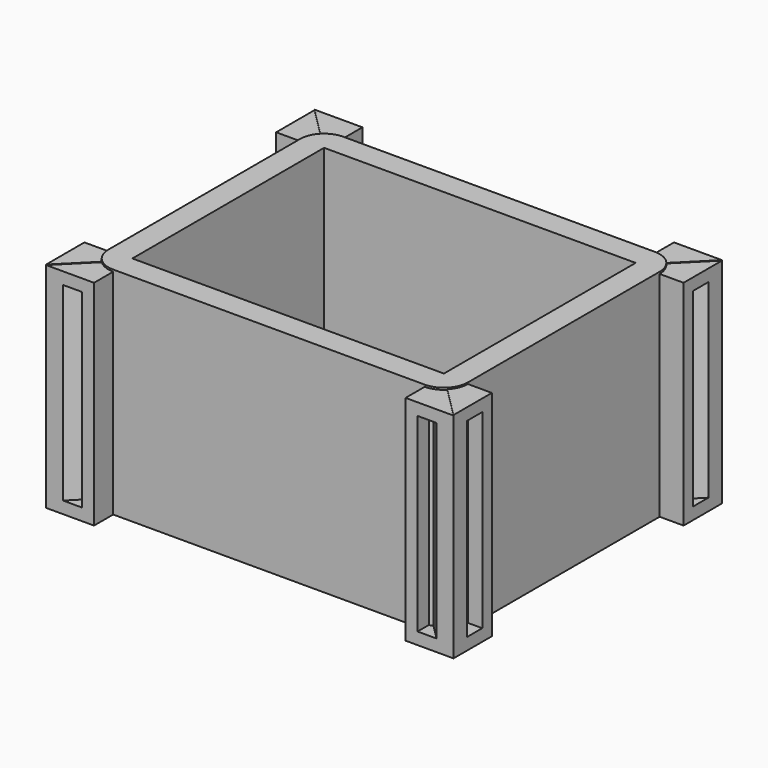
from build123d import *

# Parameters (mm, degrees)
F0_W         = 65
F0_H         = 5
F0_W_2       = 5
F0_H_2       = 50
F1_DEPTH     = 45
F2_DEPTH     = 0.1
F4_DEPTH     = 0.8
F5_DEPTH     = 44.6
F6_DEPTH     = 44.7
F7_T         = -2.5
F7_2_T       = -2.5
F7_3_T       = -2.5
F7_4_T       = -2.5
F7_5_T       = -2.5
F7_6_T       = -2.5
F7_7_T       = -2.5
F7_8_T       = -2.5
F8_TEXT_SIZE = 4.8791821529
F9_DEPTH     = 1


# Not quite as in the source:
# - Text() gives the source's letters only with a copy of the font that has no kerning and outlines rounded to 1/6400 em; it was checked with that copy


with BuildPart() as f1:
    # F0 (on Top) → F1 (new body)
    with BuildSketch(Plane.XY):
        with Locations((0, -27.5)):
            Rectangle(F0_W, F0_H)
        with Locations((0, 27.5)):
            Rectangle(F0_W, F0_H)
        with Locations((35, 0)):
            Rectangle(F0_W_2, F0_H_2)
        with Locations((-35, 0)):
            Rectangle(F0_W_2, F0_H_2)
        with BuildLine():
            Line((36.0355339059, 28.5355339059), (32.5, 25))
            Line((32.5, 25), (37.5, 25))
            ThreePointArc((37.5, 25), (37.1193976626, 26.9134171618), (36.0355339059, 28.5355339059))
        make_face()
        with BuildLine():
            Line((32.5, 30), (32.5, 25))
            Line((32.5, 25), (36.0355339059, 28.5355339059))
            ThreePointArc((36.0355339059, 28.5355339059), (34.4134171618, 29.6193976626), (32.5, 30))
        make_face()
        with BuildLine():
            Line((32.5, -25), (32.5, -30))
            ThreePointArc((32.5, -30), (34.4134171618, -29.6193976626), (36.0355339059, -28.5355339059))
            Line((36.0355339059, -28.5355339059), (32.5, -25))
        make_face()
        with BuildLine():
            Line((32.5, -25), (36.0355339059, -28.5355339059))
            ThreePointArc((36.0355339059, -28.5355339059), (37.1193976626, -26.9134171618), (37.5, -25))
            Line((37.5, -25), (32.5, -25))
        make_face()
        with BuildLine():
            ThreePointArc((-37.5, -25), (-37.1193976626, -26.9134171618), (-36.0355339059, -28.5355339059))
            Line((-36.0355339059, -28.5355339059), (-32.5, -25))
            Line((-32.5, -25), (-37.5, -25))
        make_face()
        with BuildLine():
            ThreePointArc((-36.0355339059, -28.5355339059), (-34.4134171618, -29.6193976626), (-32.5, -30))
            Line((-32.5, -30), (-32.5, -25))
            Line((-32.5, -25), (-36.0355339059, -28.5355339059))
        make_face()
        with BuildLine():
            Line((-36.0355339059, 28.5355339059), (-32.5, 25))
            Line((-32.5, 25), (-32.5, 30))
            ThreePointArc((-32.5, 30), (-34.4134171618, 29.6193976626), (-36.0355339059, 28.5355339059))
        make_face()
        with BuildLine():
            Line((-37.5, 25), (-32.5, 25))
            Line((-32.5, 25), (-36.0355339059, 28.5355339059))
            ThreePointArc((-36.0355339059, 28.5355339059), (-37.1193976626, 26.9134171618), (-37.5, 25))
        make_face()
    extrude(amount=F1_DEPTH)

    # F0 (on Top) → F2 (join)
    with BuildSketch(Plane.XY):
        Rectangle(F0_W, F0_H_2)
    extrude(amount=F2_DEPTH)

    # F3 (on face) → F4 (join)
    with BuildSketch(Plane.XY):
        Polygon((9.8419218215, 7.8486707481), (0, 12.5882904977), (-9.8419218215, 7.8486707481), (-12.2726757728, -2.8011581585), (-5.4618545502, -11.3416578385), (5.4618545502, -11.3416578385), (12.2726757728, -2.8011581585), align=None)
        Polygon((4.0130618095, 14.8103222201), (5.6598507799, 20.3949809074), (1.6467889705, 24.6134713342), (-4.0130618095, 23.2473030736), (-5.6598507799, 17.6626443863), (-1.6467889705, 13.4441539595), align=None)
        Polygon((-15.0811464459, -4.2184904268), (-13.4343574755, 1.3661682606), (-17.447419285, 5.5846586873), (-23.1072700649, 4.2184904268), (-24.7540590353, -1.3661682606), (-20.7409972259, -5.5846586873), align=None)
        Polygon((22.6341824114, -4.2184904268), (24.2809713818, 1.3661682606), (20.2679095724, 5.5846586873), (14.6080587924, 4.2184904268), (12.961269822, -1.3661682606), (16.9743316314, -5.5846586873), align=None)
        Polygon((4.0130618095, -23.7464398195), (5.6598507799, -18.1617811322), (1.6467889705, -13.9432907055), (-4.0130618095, -15.309458966), (-5.6598507799, -20.8941176534), (-1.6467889705, -25.1126080801), align=None)
    extrude(amount=F4_DEPTH)

    # F8 (on face) → F9 (join)
    with BuildSketch(Plane(origin=(0, 30, 0), x_dir=(-1, 0, 0), z_dir=(0, 1, 0))):
        with Locations((-26.7379190773, 13.3689595386)):
            Text('Vote For Harambe 2017', F8_TEXT_SIZE, font='Open Sans', text_align=(TextAlign.LEFT, TextAlign.BOTTOM))
    extrude(amount=F9_DEPTH)


with BuildPart() as f5:
    # F0 (on Top) → F5 (new body)
    with BuildSketch(Plane.XY):
        with BuildLine():
            Line((-42.5, 25), (-37.5, 25))
            ThreePointArc((-37.5, 25), (-37.1193976626, 26.9134171618), (-36.0355339059, 28.5355339059))
            Line((-36.0355339059, 28.5355339059), (-42.5, 35))
            Line((-42.5, 35), (-42.5, 25))
        make_face()
    extrude(amount=F5_DEPTH)

    # F7#8
    f7_8_openings = [f5.faces().sort_by_distance(p)[0] for p in [
        (-42.5, 30, 22.3),
    ]]
    offset(amount=F7_8_T, openings=f7_8_openings)


with BuildPart() as f5b:
    # F0 (on Top) → F5, piece 2 (new body)
    with BuildSketch(Plane.XY):
        with BuildLine():
            Line((-32.5, -35), (-32.5, -30))
            ThreePointArc((-32.5, -30), (-34.4134171618, -29.6193976626), (-36.0355339059, -28.5355339059))
            Line((-36.0355339059, -28.5355339059), (-42.5, -35))
            Line((-42.5, -35), (-32.5, -35))
        make_face()
    extrude(amount=F5_DEPTH)

    # F7
    f7_openings = [f5b.faces().sort_by_distance(p)[0] for p in [
        (-37.5, -35, 22.3),
    ]]
    offset(amount=F7_T, openings=f7_openings)


with BuildPart() as f5c:
    # F0 (on Top) → F5, piece 3 (new body)
    with BuildSketch(Plane.XY):
        with BuildLine():
            ThreePointArc((36.0355339059, 28.5355339059), (37.1193976626, 26.9134171618), (37.5, 25))
            Line((37.5, 25), (42.5, 25))
            Line((42.5, 25), (42.5, 35))
            Line((42.5, 35), (36.0355339059, 28.5355339059))
        make_face()
    extrude(amount=F5_DEPTH)

    # F7#5
    f7_5_openings = [f5c.faces().sort_by_distance(p)[0] for p in [
        (42.5, 30, 22.3),
    ]]
    offset(amount=F7_5_T, openings=f7_5_openings)


with BuildPart() as f5d:
    # F0 (on Top) → F5, piece 4 (new body)
    with BuildSketch(Plane.XY):
        with BuildLine():
            ThreePointArc((36.0355339059, -28.5355339059), (34.4134171618, -29.6193976626), (32.5, -30))
            Line((32.5, -30), (32.5, -35))
            Line((32.5, -35), (42.5, -35))
            Line((42.5, -35), (36.0355339059, -28.5355339059))
        make_face()
    extrude(amount=F5_DEPTH)

    # F7#3
    f7_3_openings = [f5d.faces().sort_by_distance(p)[0] for p in [
        (37.5, -35, 22.3),
    ]]
    offset(amount=F7_3_T, openings=f7_3_openings)


with BuildPart() as f6:
    # F0 (on Top) → F6 (new body)
    with BuildSketch(Plane.XY):
        with BuildLine():
            Line((-42.5, -35), (-36.0355339059, -28.5355339059))
            ThreePointArc((-36.0355339059, -28.5355339059), (-37.1193976626, -26.9134171618), (-37.5, -25))
            Line((-37.5, -25), (-42.5, -25))
            Line((-42.5, -25), (-42.5, -35))
        make_face()
    extrude(amount=F6_DEPTH)

    # F7#2
    f7_2_openings = [f6.faces().sort_by_distance(p)[0] for p in [
        (-42.5, -30, 22.35),
    ]]
    offset(amount=F7_2_T, openings=f7_2_openings)


with BuildPart() as f6b:
    # F0 (on Top) → F6, piece 2 (new body)
    with BuildSketch(Plane.XY):
        with BuildLine():
            ThreePointArc((37.5, -25), (37.1193976626, -26.9134171618), (36.0355339059, -28.5355339059))
            Line((36.0355339059, -28.5355339059), (42.5, -35))
            Line((42.5, -35), (42.5, -25))
            Line((42.5, -25), (37.5, -25))
        make_face()
    extrude(amount=F6_DEPTH)

    # F7#4
    f7_4_openings = [f6b.faces().sort_by_distance(p)[0] for p in [
        (42.5, -30, 22.35),
    ]]
    offset(amount=F7_4_T, openings=f7_4_openings)


with BuildPart() as f6c:
    # F0 (on Top) → F6, piece 3 (new body)
    with BuildSketch(Plane.XY):
        with BuildLine():
            Line((32.5, 35), (32.5, 30))
            ThreePointArc((32.5, 30), (34.4134171618, 29.6193976626), (36.0355339059, 28.5355339059))
            Line((36.0355339059, 28.5355339059), (42.5, 35))
            Line((42.5, 35), (32.5, 35))
        make_face()
    extrude(amount=F6_DEPTH)

    # F7#6
    f7_6_openings = [f6c.faces().sort_by_distance(p)[0] for p in [
        (37.5, 35, 22.35),
    ]]
    offset(amount=F7_6_T, openings=f7_6_openings)


with BuildPart() as f6d:
    # F0 (on Top) → F6, piece 4 (new body)
    with BuildSketch(Plane.XY):
        with BuildLine():
            ThreePointArc((-36.0355339059, 28.5355339059), (-34.4134171618, 29.6193976626), (-32.5, 30))
            Line((-32.5, 30), (-32.5, 35))
            Line((-32.5, 35), (-42.5, 35))
            Line((-42.5, 35), (-36.0355339059, 28.5355339059))
        make_face()
    extrude(amount=F6_DEPTH)

    # F7#7
    f7_7_openings = [f6d.faces().sort_by_distance(p)[0] for p in [
        (-37.5, 35, 22.35),
    ]]
    offset(amount=F7_7_T, openings=f7_7_openings)


solid = Compound([f1.part, f5.part, f5b.part, f5c.part, f5d.part, f6.part, f6b.part, f6c.part, f6d.part])
